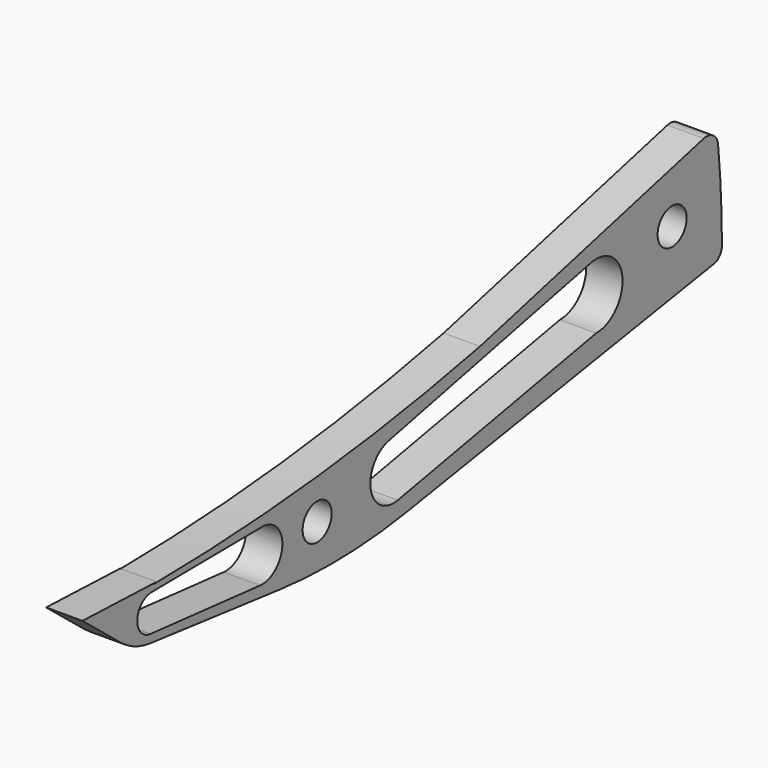
from build123d import *

# Parameters (mm, degrees)
F0_R     = 2.5
F1_DEPTH = 5


# Not quite as in the source:
# - a feature names something its author has since deleted; it is built from what else it names


with BuildPart() as f1:
    # F0 (on Right) → F1 (new body)
    with BuildSketch(Plane.YZ):
        with BuildLine():
            ThreePointArc((118.6011307413, 10.3511984734), (119.6029410321, 10.9159653279), (119.9999999073, 11.9952844227))
            ThreePointArc((119.9999999073, 11.9952844227), (119.8357295493, 18.2767765127), (119.3428752162, 24.5410579746))
            ThreePointArc((119.3428752162, 24.5410579746), (118.5020303548, 25.9696085801), (116.872434029, 26.2732411356))
            Line((116.872434029, 26.2732411356), (78.344444671, 16.7187866332))
            ThreePointArc((78.344444671, 16.7187866332), (50.4120849121, 12.3407543123), (22.1844688263, 10.7327808001))
            ThreePointArc((22.1844688263, 10.7327808001), (22.4292060309, 10.7620820299), (22.6716738588, 10.8064014821))
            Line((22.6716738588, 10.8064014821), (9.8850433167, 11.2693933781))
            Line((9.8850433167, 11.2693933781), (16.5052597895, 5.9341389572))
            ThreePointArc((16.5052597895, 5.9341389572), (18.9230306979, 4.4941821172), (21.6462541623, 3.7848543869))
            Line((21.6462541623, 3.7848543869), (43.8305606526, 1.2529498543))
            ThreePointArc((43.8305606526, 1.2529498543), (54.7908574561, 0.7592543704), (65.7156304083, 1.7697874952))
            Line((65.7156304083, 1.7697874952), (118.6011307413, 10.3511984734))
        make_face()
        with BuildLine():
            ThreePointArc((41.0425990366, 10.096905354), (44.3135999527, 6.3287058646), (40.4926591764, 3.1194713813))
            Line((40.4926591764, 3.1194713813), (21.6135530725, 4.9170973917))
            ThreePointArc((21.6135530725, 4.9170973917), (21.5948304706, 4.9188091028), (21.5761212705, 4.9206615636))
            ThreePointArc((21.5761212705, 4.9206615636), (19.3333513171, 7.4955245428), (21.7516674536, 9.9062678907))
            ThreePointArc((21.7516674536, 9.9062678907), (21.8070986498, 9.9074304985), (21.8625419965, 9.9073635786))
            Line((21.8625419965, 9.9073635786), (40.5372507264, 10.0919113847))
            ThreePointArc((40.5372507264, 10.0919113847), (40.7898346274, 10.1035413352), (41.0425990366, 10.096905354))
        make_face(mode=Mode.SUBTRACT)
        with Locations((50.3031872213, 6.8563437089)):
            Circle(F0_R, mode=Mode.SUBTRACT)
        with BuildLine():
            ThreePointArc((97.4222943066, 19.082035474), (102.8677433707, 15.1465744396), (98.3342272396, 10.1879455412))
            Line((98.3342272396, 10.1879455412), (64.1951699406, 3.8271960831))
            ThreePointArc((64.1951699406, 3.8271960831), (59.5398910648, 6.9765078631), (62.6292671904, 11.6717758272))
            Line((62.6292671904, 11.6717758272), (97.4222943066, 19.082035474))
        make_face(mode=Mode.SUBTRACT)
        with Locations((111.4225909114, 17.8264938295)):
            Circle(F0_R, mode=Mode.SUBTRACT)
    extrude(amount=F1_DEPTH)


solid = f1.part
